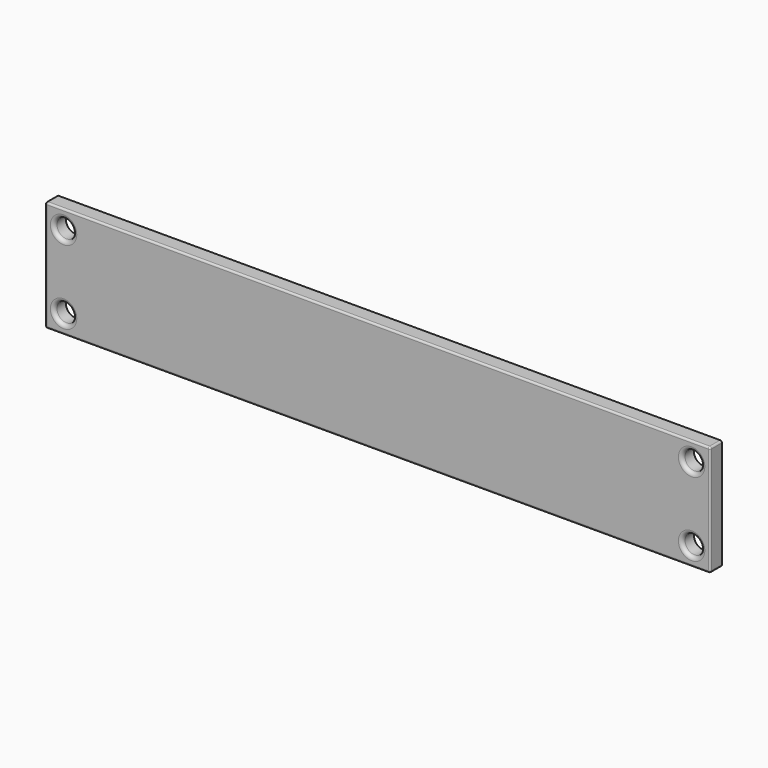
from build123d import *

# Parameters (mm, degrees)
F0_W         = 180
F0_H         = 30
F0_R         = 2.5751263091
F1_DEPTH     = 4
F2_R         = 1
F3_R         = 0.5
F4_TEXT_SIZE = 8.0589309324
F5_DEPTH     = 1


# Not quite as in the source:
# - a feature names something its author has since deleted; it is built from what else it names
# - Text() gives the source's letters only with a copy of the font that has no kerning and outlines rounded to 1/6400 em; it was checked with that copy


with BuildPart() as f1:
    # F0 (on Front) → F1 (new body)
    with BuildSketch(Plane.XZ):
        Rectangle(F0_W, F0_H)
        with Locations((-85, -10)):
            Circle(F0_R, mode=Mode.SUBTRACT)
        with Locations((85, -10)):
            Circle(F0_R, mode=Mode.SUBTRACT)
        with Locations((-85, 10)):
            Circle(F0_R, mode=Mode.SUBTRACT)
        with Locations((85, 10)):
            Circle(F0_R, mode=Mode.SUBTRACT)
    extrude(amount=F1_DEPTH)

    # F2
    f2_edges = [f1.edges().sort_by_distance(p)[0] for p in [
        (-87.575126, -4, 10),
        (-87.575126, -4, -10),
        (82.424874, -4, 10),
        (82.424874, -4, -10),
    ]]
    fillet(f2_edges, radius=F2_R)

    # F3
    f3_edges = [f1.edges().sort_by_distance(p)[0] for p in [
        (0, -4, 15),
        (-90, -4, 0),
        (0, -4, -15),
        (90, -4, 0),
        (-90, -2, 15),
        (-90, -2, -15),
        (90, -2, 15),
        (90, -2, -15),
    ]]
    fillet(f3_edges, radius=F3_R)

    # F4 (on face) → F5 (join)
    with BuildSketch(Plane(origin=(0, 0, 0), x_dir=(-1, 0, 0), z_dir=(0, 1, 0))):
        with Locations((-70.7097770646, -2.9456716736)):
            Text('Tetra Stylus Cap', F4_TEXT_SIZE, font='Open Sans', text_align=(TextAlign.LEFT, TextAlign.BOTTOM))
    extrude(amount=F5_DEPTH)

    # F6: F1 across plane


with BuildPart() as f1_1:
    add(f1.part)
    add(f1.part.mirror(Plane.YZ))


solid = f1_1.part
